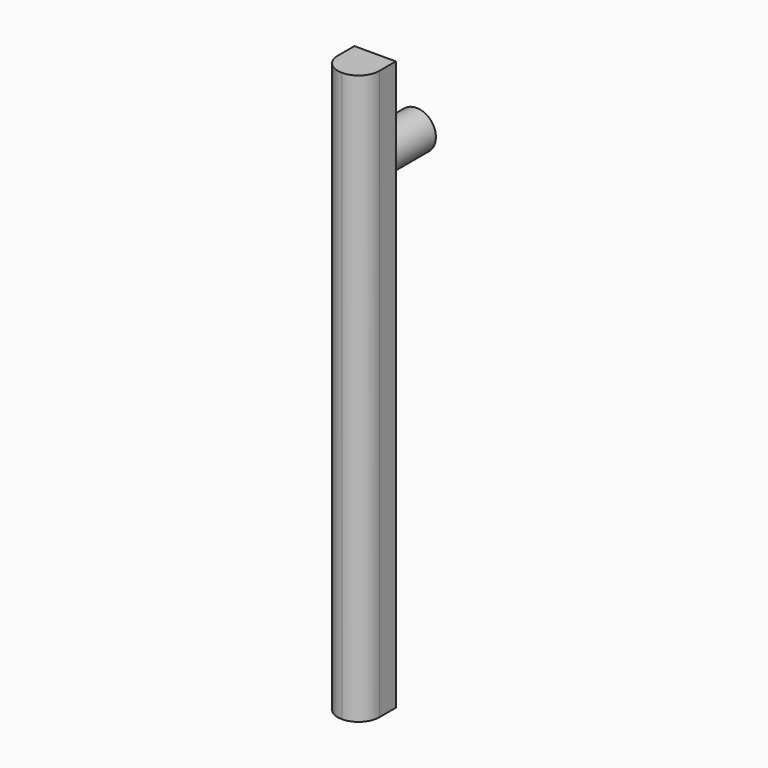
from build123d import *

# Parameters (mm, degrees)
F0_W     = 16
F0_H     = 16
F1_DEPTH = 220
F2_R     = 7.99999
F3_R     = 7.5
F4_DEPTH = 20


# Not quite as in the source:
# - a fillet or chamfer is up to 0.001 mm smaller than in the source, because OpenCascade refuses the exact size


with BuildPart() as f1:
    # F0 (on Top) → F1 (new body)
    with BuildSketch(Plane.XY):
        with Locations((-0.2842125371, -4.0679279789)):
            Rectangle(F0_W, F0_H)
    extrude(amount=F1_DEPTH)

    # F2 (radius 8 in the source; OpenCascade refuses exactly that, so slightly less here)
    f2_edges = [f1.edges().sort_by_distance(p)[0] for p in [
        (-8.284213, -12.067928, 110),
        (7.715787, -12.067928, 110),
    ]]
    fillet(f2_edges, radius=F2_R)

    # F3 (on face) → F4 (join)
    with BuildSketch(Plane(origin=(0, 3.9320720211, 0), x_dir=(-1, 0, 0), z_dir=(0, 1, 0))):
        with Locations((0.2842125371, 185.9523057938)):
            Circle(F3_R)
    extrude(amount=F4_DEPTH)


solid = f1.part
